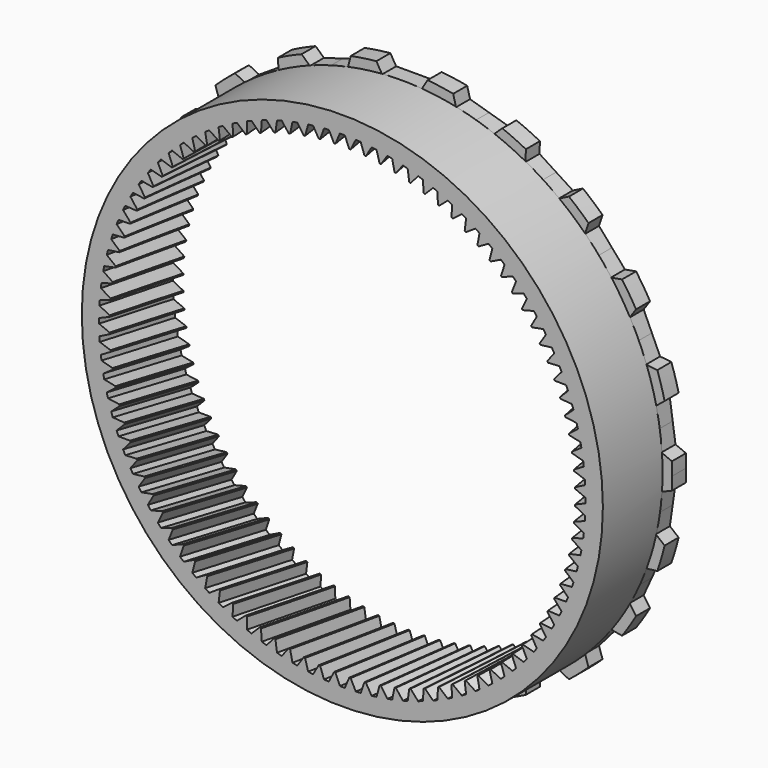
from build123d import *

# Parameters (mm, degrees)
F0_R            = 79.3242
F1_DEPTH        = 5.969
F2_R            = 88.773
F2_R_2          = 79.3242
F3_DEPTH        = 25.4
F8_COPIES_COUNT = 96


# Not quite as in the source:
# - a pattern or mirror of a feature is missing from the dataset's text; its kind, count and spacing are read off the source's solid


with BuildPart() as f1:
    # F0 (on Front) → F1 (new body)
    with BuildSketch(Plane.XZ):
        with BuildLine():
            ThreePointArc((91.9693972023, -4.4085829063), (92.0485955146, -2.2049237624), (92.075, 0))
            ThreePointArc((92.075, 0), (92.0485955146, 2.2049237624), (91.9693972023, 4.4085829063))
            Line((91.9693972023, 4.4085829063), (88.4190526436, 5.899693551))
            Line((88.4190526436, 5.899693551), (87.4593240688, 12.5747524086))
            Line((87.4593240688, 12.5747524086), (86.4995954939, 19.2498112662))
            Line((86.4995954939, 19.2498112662), (89.4860317374, 21.6807691028))
            ThreePointArc((89.4860317374, 21.6807691028), (88.3453155456, 25.9405251712), (87.001949069, 30.1407777471))
            Line((87.001949069, 30.1407777471), (83.1753239965, 30.5712402834))
            Line((83.1753239965, 30.5712402834), (80.3738897734, 36.7055255705))
            Line((80.3738897734, 36.7055255705), (77.5724555502, 42.8398108576))
            Line((77.5724555502, 42.8398108576), (79.7530401751, 46.0136741397))
            ThreePointArc((79.7530401751, 46.0136741397), (77.4584190354, 49.7795032672), (74.9861204425, 53.431146029))
            Line((74.9861204425, 53.431146029), (71.1932252619, 52.7660869423))
            Line((71.1932252619, 52.7660869423), (66.7770409304, 57.8626353468))
            Line((66.7770409304, 57.8626353468), (62.3608565989, 62.9591837514))
            Line((62.3608565989, 62.9591837514), (63.5589316073, 66.6188249516))
            ThreePointArc((63.5589316073, 66.6188249516), (60.296302078, 69.5856420587), (56.8953622975, 72.3928406269))
            Line((56.8953622975, 72.3928406269), (53.443474819, 70.6861390491))
            Line((53.443474819, 70.6861390491), (47.7703133697, 74.3320585297))
            Line((47.7703133697, 74.3320585297), (42.0971519203, 77.9779780104))
            Line((42.0971519203, 77.9779780104), (42.2156564003, 81.8269147634))
            ThreePointArc((42.2156564003, 81.8269147634), (38.2493373221, 83.7543659723), (34.1952802689, 85.489697814))
            Line((34.1952802689, 85.489697814), (31.3640518868, 82.8796205568))
            Line((31.3640518868, 82.8796205568), (24.8935191207, 84.7795404003))
            Line((24.8935191207, 84.7795404003), (18.4229863545, 86.6794602439))
            Line((18.4229863545, 86.6794602439), (17.4523197779, 90.4058745844))
            ThreePointArc((17.4523197779, 90.4058745844), (13.103638734, 91.1378092612), (8.7249, 91.660688111))
            Line((8.7249, 91.660688111), (6.7437, 88.358688111))
            Line((6.7437, 88.358688111), (0, 88.358688111))
            Line((0, 88.358688111), (-6.7437, 88.358688111))
            Line((-6.7437, 88.358688111), (-8.7249, 91.660688111))
            ThreePointArc((-8.7249, 91.660688111), (-13.103638734, 91.1378092612), (-17.4523197779, 90.4058745844))
            Line((-17.4523197779, 90.4058745844), (-18.4229863545, 86.6794602439))
            Line((-18.4229863545, 86.6794602439), (-24.8935191207, 84.7795404003))
            Line((-24.8935191207, 84.7795404003), (-31.3640518868, 82.8796205568))
            Line((-31.3640518868, 82.8796205568), (-34.1952802689, 85.489697814))
            ThreePointArc((-34.1952802689, 85.489697814), (-38.2493373221, 83.7543659723), (-42.2156564003, 81.8269147634))
            Line((-42.2156564003, 81.8269147634), (-42.0971519203, 77.9779780104))
            Line((-42.0971519203, 77.9779780104), (-47.7703133697, 74.3320585297))
            Line((-47.7703133697, 74.3320585297), (-53.443474819, 70.6861390491))
            Line((-53.443474819, 70.6861390491), (-56.8953622975, 72.3928406269))
            ThreePointArc((-56.8953622975, 72.3928406269), (-60.296302078, 69.5856420587), (-63.5589316073, 66.6188249516))
            Line((-63.5589316073, 66.6188249516), (-62.3608565989, 62.9591837514))
            Line((-62.3608565989, 62.9591837514), (-66.7770409304, 57.8626353468))
            Line((-66.7770409304, 57.8626353468), (-71.1932252619, 52.7660869423))
            Line((-71.1932252619, 52.7660869423), (-74.9861204425, 53.431146029))
            ThreePointArc((-74.9861204425, 53.431146029), (-77.4584190354, 49.7795032672), (-79.7530401751, 46.0136741397))
            Line((-79.7530401751, 46.0136741397), (-77.5724555502, 42.8398108576))
            Line((-77.5724555502, 42.8398108576), (-80.3738897734, 36.7055255705))
            Line((-80.3738897734, 36.7055255705), (-83.1753239965, 30.5712402834))
            Line((-83.1753239965, 30.5712402834), (-87.001949069, 30.1407777471))
            ThreePointArc((-87.001949069, 30.1407777471), (-88.3453155456, 25.9405251712), (-89.4860317374, 21.6807691028))
            Line((-89.4860317374, 21.6807691028), (-86.4995954939, 19.2498112662))
            Line((-86.4995954939, 19.2498112662), (-87.4593240688, 12.5747524086))
            Line((-87.4593240688, 12.5747524086), (-88.4190526436, 5.899693551))
            Line((-88.4190526436, 5.899693551), (-91.9693972023, 4.4085829063))
            ThreePointArc((-91.9693972023, 4.4085829063), (-92.075, 0), (-91.9693972023, -4.4085829063))
            Line((-91.9693972023, -4.4085829063), (-88.4190526436, -5.899693551))
            Line((-88.4190526436, -5.899693551), (-87.4593240688, -12.5747524086))
            Line((-87.4593240688, -12.5747524086), (-86.4995954939, -19.2498112662))
            Line((-86.4995954939, -19.2498112662), (-89.4860317374, -21.6807691028))
            ThreePointArc((-89.4860317374, -21.6807691028), (-88.3453155456, -25.9405251712), (-87.001949069, -30.1407777471))
            Line((-87.001949069, -30.1407777471), (-83.1753239965, -30.5712402834))
            Line((-83.1753239965, -30.5712402834), (-80.3738897734, -36.7055255705))
            Line((-80.3738897734, -36.7055255705), (-77.5724555502, -42.8398108576))
            Line((-77.5724555502, -42.8398108576), (-79.7530401751, -46.0136741397))
            ThreePointArc((-79.7530401751, -46.0136741397), (-77.4584190354, -49.7795032672), (-74.9861204425, -53.431146029))
            Line((-74.9861204425, -53.431146029), (-71.1932252619, -52.7660869423))
            Line((-71.1932252619, -52.7660869423), (-66.7770409304, -57.8626353468))
            Line((-66.7770409304, -57.8626353468), (-62.3608565989, -62.9591837514))
            Line((-62.3608565989, -62.9591837514), (-63.5589316073, -66.6188249516))
            ThreePointArc((-63.5589316073, -66.6188249516), (-60.296302078, -69.5856420587), (-56.8953622975, -72.3928406269))
            Line((-56.8953622975, -72.3928406269), (-53.443474819, -70.6861390491))
            Line((-53.443474819, -70.6861390491), (-47.7703133697, -74.3320585297))
            Line((-47.7703133697, -74.3320585297), (-42.0971519203, -77.9779780104))
            Line((-42.0971519203, -77.9779780104), (-42.2156564003, -81.8269147634))
            ThreePointArc((-42.2156564003, -81.8269147634), (-38.2493373221, -83.7543659723), (-34.1952802689, -85.489697814))
            Line((-34.1952802689, -85.489697814), (-31.3640518868, -82.8796205568))
            Line((-31.3640518868, -82.8796205568), (-24.8935191207, -84.7795404003))
            Line((-24.8935191207, -84.7795404003), (-18.4229863545, -86.6794602439))
            Line((-18.4229863545, -86.6794602439), (-17.4523197779, -90.4058745844))
            ThreePointArc((-17.4523197779, -90.4058745844), (-13.103638734, -91.1378092612), (-8.7249, -91.660688111))
            Line((-8.7249, -91.660688111), (-6.7437, -88.358688111))
            Line((-6.7437, -88.358688111), (0, -88.358688111))
            Line((0, -88.358688111), (6.7437, -88.358688111))
            Line((6.7437, -88.358688111), (8.7249, -91.660688111))
            ThreePointArc((8.7249, -91.660688111), (13.103638734, -91.1378092612), (17.4523197779, -90.4058745844))
            Line((17.4523197779, -90.4058745844), (18.4229863545, -86.6794602439))
            Line((18.4229863545, -86.6794602439), (24.8935191207, -84.7795404003))
            Line((24.8935191207, -84.7795404003), (31.3640518868, -82.8796205568))
            Line((31.3640518868, -82.8796205568), (34.1952802689, -85.489697814))
            ThreePointArc((34.1952802689, -85.489697814), (38.2493373221, -83.7543659723), (42.2156564003, -81.8269147634))
            Line((42.2156564003, -81.8269147634), (42.0971519203, -77.9779780104))
            Line((42.0971519203, -77.9779780104), (47.7703133697, -74.3320585297))
            Line((47.7703133697, -74.3320585297), (53.443474819, -70.6861390491))
            Line((53.443474819, -70.6861390491), (56.8953622975, -72.3928406269))
            ThreePointArc((56.8953622975, -72.3928406269), (60.296302078, -69.5856420587), (63.5589316073, -66.6188249516))
            Line((63.5589316073, -66.6188249516), (62.3608565989, -62.9591837514))
            Line((62.3608565989, -62.9591837514), (66.7770409304, -57.8626353468))
            Line((66.7770409304, -57.8626353468), (71.1932252619, -52.7660869423))
            Line((71.1932252619, -52.7660869423), (74.9861204425, -53.431146029))
            ThreePointArc((74.9861204425, -53.431146029), (77.4584190354, -49.7795032672), (79.7530401751, -46.0136741397))
            Line((79.7530401751, -46.0136741397), (77.5724555502, -42.8398108576))
            Line((77.5724555502, -42.8398108576), (80.3738897734, -36.7055255705))
            Line((80.3738897734, -36.7055255705), (83.1753239965, -30.5712402834))
            Line((83.1753239965, -30.5712402834), (87.001949069, -30.1407777471))
            ThreePointArc((87.001949069, -30.1407777471), (88.3453155456, -25.9405251712), (89.4860317374, -21.6807691028))
            Line((89.4860317374, -21.6807691028), (86.4995954939, -19.2498112662))
            Line((86.4995954939, -19.2498112662), (87.4593240688, -12.5747524086))
            Line((87.4593240688, -12.5747524086), (88.4190526436, -5.899693551))
            Line((88.4190526436, -5.899693551), (91.9693972023, -4.4085829063))
        make_face()
        Circle(F0_R, mode=Mode.SUBTRACT)
    extrude(amount=-F1_DEPTH)

    # F2 (on Front) → F3 (join)
    with BuildSketch(Plane.XZ):
        Circle(F2_R)
        Circle(F2_R_2, mode=Mode.SUBTRACT)
    extrude(amount=F3_DEPTH)

    # F8: sweep along a path in F7
    with BuildLine(Plane(origin=(0, 0.5902941867, 82.6904269589), x_dir=(1, 0, 0), z_dir=(0, -0.0071384218, -0.9999745211))) as f8_path:
        Line((-0.8382, 25.9909564065), (-6.1456817891, -5.3788428601))
    # F4 (on face) → F8 (sweep, cut)
    with BuildSketch(Plane.XZ.offset(25.4)):
        with BuildLine():
            Line((3.1078436502, 77.5340464381), (2.3622, 79.2890201529))
            ThreePointArc((2.3622, 79.2890201529), (0, 79.3242), (-2.3622, 79.2890201529))
            Line((-2.3622, 79.2890201529), (-3.1078436502, 77.5340464381))
            Line((-3.1078436502, 77.5340464381), (3.1078436502, 77.5340464381))
        make_face()
        with BuildLine():
            Line((2.3622, 79.2890201529), (0.8382, 82.8759613688))
            ThreePointArc((0.8382, 82.8759613688), (0, 82.8802), (-0.8382, 82.8759613688))
            Line((-0.8382, 82.8759613688), (-2.3622, 79.2890201529))
            ThreePointArc((-2.3622, 79.2890201529), (0, 79.3242), (2.3622, 79.2890201529))
        make_face()
    f8 = sweep(path=f8_path.line, mode=Mode.SUBTRACT)

    # F8_copies: F8 ×96 about axis
    f8_copies_axis = Axis((0, 0, 0), (0, 1, 0))
    for i in range(1, F8_COPIES_COUNT):
        add(f8.rotate(f8_copies_axis, i * 360 / F8_COPIES_COUNT), mode=Mode.SUBTRACT)


solid = f1.part
